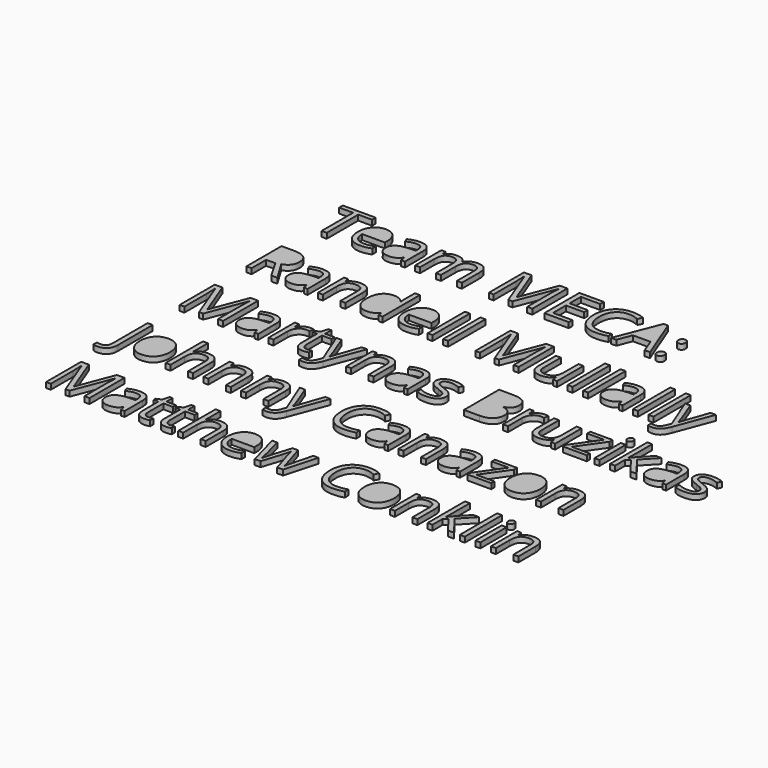
from build123d import *

# Parameters (mm, degrees)
F0_TEXT_SIZE = 6.9151809833
F1_DEPTH     = 0.6


# Not quite as in the source:
# - Text() gives the source's letters only with a copy of the font that has no kerning and outlines rounded to 1/6400 em; it was checked with that copy


with BuildPart() as f1:
    # F0 (on Top) → F1 (new body)
    with BuildSketch(Plane.XY):
        with BuildLine():
            add(Edge.make_bspline(
                [(5.8827660724, 1.8456028601), (5.6023770935, 1.484176604), (5.6023770935, 0.768887571)],
                knots=[0, 0, 0, 1, 1, 1], degree=2))
            add(Edge.make_bspline(
                [(5.6023770935, 0.768887571), (5.6023770935, 0.0590010232), (5.8860075635, -0.3121497061)],
                knots=[0, 0, 0, 1, 1, 1], degree=2))
            add(Edge.make_bspline(
                [(5.8860075635, -0.3121497061), (6.1696380335, -0.6833004355), (6.7196110211, -0.6833004355)],
                knots=[0, 0, 0, 1, 1, 1], degree=2))
            add(Edge.make_bspline(
                [(6.7196110211, -0.6833004355), (7.2706645057, -0.6833004355), (7.5559157212, -0.3137704517)],
                knots=[0, 0, 0, 1, 1, 1], degree=2))
            add(Edge.make_bspline(
                [(7.5559157212, -0.3137704517), (7.8411669368, 0.0557595321), (7.8411669368, 0.768887571)],
                knots=[0, 0, 0, 1, 1, 1], degree=2))
            add(Edge.make_bspline(
                [(7.8411669368, 0.768887571), (7.8411669368, 1.4744521307), (7.5559157212, 1.8407406234)],
                knots=[0, 0, 0, 1, 1, 1], degree=2))
            add(Edge.make_bspline(
                [(7.5559157212, 1.8407406234), (7.2706645057, 2.2070291161), (6.7131280389, 2.2070291161)],
                knots=[0, 0, 0, 1, 1, 1], degree=2))
            add(Edge.make_bspline(
                [(6.7131280389, 2.2070291161), (6.1631550513, 2.2070291161), (5.8827660724, 1.8456028601)],
                knots=[0, 0, 0, 1, 1, 1], degree=2))
        make_face()
        with BuildLine():
            add(Edge.make_bspline(
                [(14.8206374932, 11.2502489973), (14.5402485143, 10.8888227412), (14.5402485143, 10.1735337082)],
                knots=[0, 0, 0, 1, 1, 1], degree=2))
            add(Edge.make_bspline(
                [(14.5402485143, 10.1735337082), (14.5402485143, 9.4636471604), (14.8238789843, 9.0924964311)],
                knots=[0, 0, 0, 1, 1, 1], degree=2))
            add(Edge.make_bspline(
                [(14.8238789843, 9.0924964311), (15.1075094543, 8.7213457018), (15.6574824419, 8.7213457018)],
                knots=[0, 0, 0, 1, 1, 1], degree=2))
            add(Edge.make_bspline(
                [(15.6574824419, 8.7213457018), (16.2085359265, 8.7213457018), (16.4937871421, 9.0908756856)],
                knots=[0, 0, 0, 1, 1, 1], degree=2))
            add(Edge.make_bspline(
                [(16.4937871421, 9.0908756856), (16.7790383576, 9.4604056693), (16.7790383576, 10.1735337082)],
                knots=[0, 0, 0, 1, 1, 1], degree=2))
            add(Edge.make_bspline(
                [(16.7790383576, 10.1735337082), (16.7790383576, 10.8790982679), (16.4937871421, 11.2453867606)],
                knots=[0, 0, 0, 1, 1, 1], degree=2))
            add(Edge.make_bspline(
                [(16.4937871421, 11.2453867606), (16.2085359265, 11.6116752534), (15.6509994598, 11.6116752534)],
                knots=[0, 0, 0, 1, 1, 1], degree=2))
            add(Edge.make_bspline(
                [(15.6509994598, 11.6116752534), (15.1010264722, 11.6116752534), (14.8206374932, 11.2502489973)],
                knots=[0, 0, 0, 1, 1, 1], degree=2))
        make_face()
        with BuildLine():
            add(Edge.make_bspline(
                [(-26.9038357645, 11.2502489973), (-27.1842247434, 10.8888227412), (-27.1842247434, 10.1735337082)],
                knots=[0, 0, 0, 1, 1, 1], degree=2))
            add(Edge.make_bspline(
                [(-27.1842247434, 10.1735337082), (-27.1842247434, 9.4636471604), (-26.9005942734, 9.0924964311)],
                knots=[0, 0, 0, 1, 1, 1], degree=2))
            add(Edge.make_bspline(
                [(-26.9005942734, 9.0924964311), (-26.6169638033, 8.7213457018), (-26.0669908158, 8.7213457018)],
                knots=[0, 0, 0, 1, 1, 1], degree=2))
            add(Edge.make_bspline(
                [(-26.0669908158, 8.7213457018), (-25.5159373312, 8.7213457018), (-25.2306861156, 9.0908756856)],
                knots=[0, 0, 0, 1, 1, 1], degree=2))
            add(Edge.make_bspline(
                [(-25.2306861156, 9.0908756856), (-24.9454349001, 9.4604056693), (-24.9454349001, 10.1735337082)],
                knots=[0, 0, 0, 1, 1, 1], degree=2))
            add(Edge.make_bspline(
                [(-24.9454349001, 10.1735337082), (-24.9454349001, 10.8790982679), (-25.2306861156, 11.2453867606)],
                knots=[0, 0, 0, 1, 1, 1], degree=2))
            add(Edge.make_bspline(
                [(-25.2306861156, 11.2453867606), (-25.5159373312, 11.6116752534), (-26.0734737979, 11.6116752534)],
                knots=[0, 0, 0, 1, 1, 1], degree=2))
            add(Edge.make_bspline(
                [(-26.0734737979, 11.6116752534), (-26.6234467855, 11.6116752534), (-26.9038357645, 11.2502489973)],
                knots=[0, 0, 0, 1, 1, 1], degree=2))
        make_face()
        with BuildLine():
            add(Edge.make_bspline(
                [(-16.4068071313, 27.8920642323), (-16.1469475959, 27.5306379762), (-15.6434359806, 27.5306379762)],
                knots=[0, 0, 0, 1, 1, 1], degree=2))
            add(Edge.make_bspline(
                [(-15.6434359806, 27.5306379762), (-15.0696920583, 27.5306379762), (-14.8114532685, 27.8429016175)],
                knots=[0, 0, 0, 1, 1, 1], degree=2))
            add(Edge.make_bspline(
                [(-14.8114532685, 27.8429016175), (-14.5532144787, 28.1551652588), (-14.5532144787, 28.8510053452)],
                knots=[0, 0, 0, 1, 1, 1], degree=2))
            Line((-14.5532144787, 28.8510053452), (-14.5532144787, 28.9687795213))
            add(Edge.make_bspline(
                [(-14.5532144787, 28.9687795213), (-14.5532144787, 29.7553813582), (-14.8146947596, 30.0914159341)],
                knots=[0, 0, 0, 1, 1, 1], degree=2))
            add(Edge.make_bspline(
                [(-14.8146947596, 30.0914159341), (-15.0761750405, 30.42745051), (-15.6499189627, 30.42745051)],
                knots=[0, 0, 0, 1, 1, 1], degree=2))
            add(Edge.make_bspline(
                [(-15.6499189627, 30.42745051), (-16.1437061048, 30.42745051), (-16.4051863857, 30.0444143133)],
                knots=[0, 0, 0, 1, 1, 1], degree=2))
            add(Edge.make_bspline(
                [(-16.4051863857, 30.0444143133), (-16.6666666667, 29.6613781167), (-16.6666666667, 28.9622965391)],
                knots=[0, 0, 0, 1, 1, 1], degree=2))
            add(Edge.make_bspline(
                [(-16.6666666667, 28.9622965391), (-16.6666666667, 28.2534904884), (-16.4068071313, 27.8920642323)],
                knots=[0, 0, 0, 1, 1, 1], degree=2))
        make_face()
        with Locations((-30, 8.3194008071)):
            Text('Johnny Canazon', F0_TEXT_SIZE, font='Open Sans', text_align=(TextAlign.LEFT, TextAlign.BOTTOM))
        with BuildLine():
            Line((4.2582387898, 20.0611620173), (3.2749864938, 20.0611620173))
            Line((3.2749864938, 20.0611620173), (3.2749864938, 18.2135120983))
            Line((3.2749864938, 18.2135120983), (4.3057806591, 18.2135120983))
            add(Edge.make_bspline(
                [(4.3057806591, 18.2135120983), (4.9032955159, 18.2135120983), (5.2052944354, 18.4447384624)],
                knots=[0, 0, 0, 1, 1, 1], degree=2))
            add(Edge.make_bspline(
                [(5.2052944354, 18.4447384624), (5.5072933549, 18.6759648266), (5.5072933549, 19.1697519686)],
                knots=[0, 0, 0, 1, 1, 1], degree=2))
            add(Edge.make_bspline(
                [(5.5072933549, 19.1697519686), (5.5072933549, 19.6289632058), (5.1982712048, 19.8450626115)],
                knots=[0, 0, 0, 1, 1, 1], degree=2))
            add(Edge.make_bspline(
                [(5.1982712048, 19.8450626115), (4.8892490546, 20.0611620173), (4.2582387898, 20.0611620173)],
                knots=[0, 0, 0, 1, 1, 1], degree=2))
        make_face()
        with BuildLine():
            Line((-28.7477039438, 31.56197239), (-28.7477039438, 29.674344081))
            Line((-28.7477039438, 29.674344081), (-27.9600216099, 29.674344081))
            add(Edge.make_bspline(
                [(-27.9600216099, 29.674344081), (-27.3527822798, 29.674344081), (-27.0691518098, 29.9158351669)],
                knots=[0, 0, 0, 1, 1, 1], degree=2))
            add(Edge.make_bspline(
                [(-27.0691518098, 29.9158351669), (-26.7855213398, 30.1573262528), (-26.7855213398, 30.6403084246)],
                knots=[0, 0, 0, 1, 1, 1], degree=2))
            add(Edge.make_bspline(
                [(-26.7855213398, 30.6403084246), (-26.7855213398, 31.1297735786), (-27.0740140465, 31.3458729843)],
                knots=[0, 0, 0, 1, 1, 1], degree=2))
            add(Edge.make_bspline(
                [(-27.0740140465, 31.3458729843), (-27.3625067531, 31.56197239), (-28.001080497, 31.56197239)],
                knots=[0, 0, 0, 1, 1, 1], degree=2))
            Line((-28.001080497, 31.56197239), (-28.7477039438, 31.56197239))
        make_face()
        with BuildLine():
            Line((3.2749864938, 22.163809235), (3.2749864938, 20.5473856802))
            Line((3.2749864938, 20.5473856802), (4.2204213938, 20.5473856802))
            add(Edge.make_bspline(
                [(4.2204213938, 20.5473856802), (4.828741221, 20.5473856802), (5.095623987, 20.7380934057)],
                knots=[0, 0, 0, 1, 1, 1], degree=2))
            add(Edge.make_bspline(
                [(5.095623987, 20.7380934057), (5.3625067531, 20.9288011313), (5.3625067531, 21.3804488892)],
                knots=[0, 0, 0, 1, 1, 1], degree=2))
            add(Edge.make_bspline(
                [(5.3625067531, 21.3804488892), (5.3625067531, 21.7964402453), (5.0653700702, 21.9801247401)],
                knots=[0, 0, 0, 1, 1, 1], degree=2))
            add(Edge.make_bspline(
                [(5.0653700702, 21.9801247401), (4.7682333874, 22.163809235), (4.1199351702, 22.163809235)],
                knots=[0, 0, 0, 1, 1, 1], degree=2))
            Line((4.1199351702, 22.163809235), (3.2749864938, 22.163809235))
        make_face()
        with Locations((-30, 27.1286930816)):
            Text('Randell Mullally', F0_TEXT_SIZE, font='Open Sans', text_align=(TextAlign.LEFT, TextAlign.BOTTOM))
        with BuildLine():
            add(Edge.make_bspline(
                [(-21.2047541869, 37.087093946), (-21.0210696921, 36.9288011313), (-20.6904376013, 36.9288011313)],
                knots=[0, 0, 0, 1, 1, 1], degree=2))
            add(Edge.make_bspline(
                [(-20.6904376013, 36.9288011313), (-20.1663965424, 36.9288011313), (-19.867639114, 37.2156730924)],
                knots=[0, 0, 0, 1, 1, 1], degree=2))
            add(Edge.make_bspline(
                [(-19.867639114, 37.2156730924), (-19.5688816856, 37.5025450535), (-19.5688816856, 38.0190226331)],
                knots=[0, 0, 0, 1, 1, 1], degree=2))
            Line((-19.5688816856, 38.0190226331), (-19.5688816856, 38.352896215))
            Line((-19.5688816856, 38.352896215), (-20.1296596434, 38.3302057774))
            add(Edge.make_bspline(
                [(-20.1296596434, 38.3302057774), (-20.7984873042, 38.3064348428), (-21.093462993, 38.1222100994)],
                knots=[0, 0, 0, 1, 1, 1], degree=2))
            add(Edge.make_bspline(
                [(-21.093462993, 38.1222100994), (-21.3884386818, 37.937985356), (-21.3884386818, 37.5500869227)],
                knots=[0, 0, 0, 1, 1, 1], degree=2))
            add(Edge.make_bspline(
                [(-21.3884386818, 37.5500869227), (-21.3884386818, 37.2453867606), (-21.2047541869, 37.087093946)],
                knots=[0, 0, 0, 1, 1, 1], degree=2))
        make_face()
        with BuildLine():
            add(Edge.make_bspline(
                [(-24.6364127499, 27.6824478087), (-24.452728255, 27.524154994), (-24.1220961642, 27.524154994)],
                knots=[0, 0, 0, 1, 1, 1], degree=2))
            add(Edge.make_bspline(
                [(-24.1220961642, 27.524154994), (-23.5980551053, 27.524154994), (-23.2992976769, 27.8110269551)],
                knots=[0, 0, 0, 1, 1, 1], degree=2))
            add(Edge.make_bspline(
                [(-23.2992976769, 27.8110269551), (-23.0005402485, 28.0978989162), (-23.0005402485, 28.6143764959)],
                knots=[0, 0, 0, 1, 1, 1], degree=2))
            Line((-23.0005402485, 28.6143764959), (-23.0005402485, 28.9482500778))
            Line((-23.0005402485, 28.9482500778), (-23.5613182064, 28.9255596402))
            add(Edge.make_bspline(
                [(-23.5613182064, 28.9255596402), (-24.2301458671, 28.9017887055), (-24.5251215559, 28.7175639622)],
                knots=[0, 0, 0, 1, 1, 1], degree=2))
            add(Edge.make_bspline(
                [(-24.5251215559, 28.7175639622), (-24.8200972447, 28.5333392188), (-24.8200972447, 28.1454407855)],
                knots=[0, 0, 0, 1, 1, 1], degree=2))
            add(Edge.make_bspline(
                [(-24.8200972447, 28.1454407855), (-24.8200972447, 27.8407406234), (-24.6364127499, 27.6824478087)],
                knots=[0, 0, 0, 1, 1, 1], degree=2))
        make_face()
        with BuildLine():
            add(Edge.make_bspline(
                [(10.8525121556, 27.6824478087), (11.0361966505, 27.524154994), (11.3668287412, 27.524154994)],
                knots=[0, 0, 0, 1, 1, 1], degree=2))
            add(Edge.make_bspline(
                [(11.3668287412, 27.524154994), (11.8908698001, 27.524154994), (12.1896272285, 27.8110269551)],
                knots=[0, 0, 0, 1, 1, 1], degree=2))
            add(Edge.make_bspline(
                [(12.1896272285, 27.8110269551), (12.4883846569, 28.0978989162), (12.4883846569, 28.6143764959)],
                knots=[0, 0, 0, 1, 1, 1], degree=2))
            Line((12.4883846569, 28.6143764959), (12.4883846569, 28.9482500778))
            Line((12.4883846569, 28.9482500778), (11.9276066991, 28.9255596402))
            add(Edge.make_bspline(
                [(11.9276066991, 28.9255596402), (11.2587790384, 28.9017887055), (10.9638033495, 28.7175639622)],
                knots=[0, 0, 0, 1, 1, 1], degree=2))
            add(Edge.make_bspline(
                [(10.9638033495, 28.7175639622), (10.6688276607, 28.5333392188), (10.6688276607, 28.1454407855)],
                knots=[0, 0, 0, 1, 1, 1], degree=2))
            add(Edge.make_bspline(
                [(10.6688276607, 28.1454407855), (10.6688276607, 27.8407406234), (10.8525121556, 27.6824478087)],
                knots=[0, 0, 0, 1, 1, 1], degree=2))
        make_face()
        with BuildLine():
            add(Edge.make_bspline(
                [(-22.6677471637, 18.2778016715), (-22.4840626688, 18.1195088568), (-22.1534305781, 18.1195088568)],
                knots=[0, 0, 0, 1, 1, 1], degree=2))
            add(Edge.make_bspline(
                [(-22.1534305781, 18.1195088568), (-21.6293895192, 18.1195088568), (-21.3306320908, 18.4063808179)],
                knots=[0, 0, 0, 1, 1, 1], degree=2))
            add(Edge.make_bspline(
                [(-21.3306320908, 18.4063808179), (-21.0318746623, 18.693252779), (-21.0318746623, 19.2097303587)],
                knots=[0, 0, 0, 1, 1, 1], degree=2))
            Line((-21.0318746623, 19.2097303587), (-21.0318746623, 19.5436039406))
            Line((-21.0318746623, 19.5436039406), (-21.5926526202, 19.5209135029))
            add(Edge.make_bspline(
                [(-21.5926526202, 19.5209135029), (-22.2614802809, 19.4971425683), (-22.5564559697, 19.3129178249)],
                knots=[0, 0, 0, 1, 1, 1], degree=2))
            add(Edge.make_bspline(
                [(-22.5564559697, 19.3129178249), (-22.8514316586, 19.1286930816), (-22.8514316586, 18.7407946483)],
                knots=[0, 0, 0, 1, 1, 1], degree=2))
            add(Edge.make_bspline(
                [(-22.8514316586, 18.7407946483), (-22.8514316586, 18.4360944862), (-22.6677471637, 18.2778016715)],
                knots=[0, 0, 0, 1, 1, 1], degree=2))
        make_face()
        with BuildLine():
            add(Edge.make_bspline(
                [(-5.8292814695, 18.2778016715), (-5.6455969746, 18.1195088568), (-5.3149648838, 18.1195088568)],
                knots=[0, 0, 0, 1, 1, 1], degree=2))
            add(Edge.make_bspline(
                [(-5.3149648838, 18.1195088568), (-4.790923825, 18.1195088568), (-4.4921663965, 18.4063808179)],
                knots=[0, 0, 0, 1, 1, 1], degree=2))
            add(Edge.make_bspline(
                [(-4.4921663965, 18.4063808179), (-4.1934089681, 18.693252779), (-4.1934089681, 19.2097303587)],
                knots=[0, 0, 0, 1, 1, 1], degree=2))
            Line((-4.1934089681, 19.2097303587), (-4.1934089681, 19.5436039406))
            Line((-4.1934089681, 19.5436039406), (-4.754186926, 19.5209135029))
            add(Edge.make_bspline(
                [(-4.754186926, 19.5209135029), (-5.4230145867, 19.4971425683), (-5.7179902755, 19.3129178249)],
                knots=[0, 0, 0, 1, 1, 1], degree=2))
            add(Edge.make_bspline(
                [(-5.7179902755, 19.3129178249), (-6.0129659643, 19.1286930816), (-6.0129659643, 18.7407946483)],
                knots=[0, 0, 0, 1, 1, 1], degree=2))
            add(Edge.make_bspline(
                [(-6.0129659643, 18.7407946483), (-6.0129659643, 18.4360944862), (-5.8292814695, 18.2778016715)],
                knots=[0, 0, 0, 1, 1, 1], degree=2))
        make_face()
        with BuildLine():
            add(Edge.make_bspline(
                [(-0.5099945975, 8.8731555343), (-0.3263101026, 8.7148627196), (0.0043219881, 8.7148627196)],
                knots=[0, 0, 0, 1, 1, 1], degree=2))
            add(Edge.make_bspline(
                [(0.0043219881, 8.7148627196), (0.528363047, 8.7148627196), (0.8271204754, 9.0017346807)],
                knots=[0, 0, 0, 1, 1, 1], degree=2))
            add(Edge.make_bspline(
                [(0.8271204754, 9.0017346807), (1.1258779038, 9.2886066418), (1.1258779038, 9.8050842215)],
                knots=[0, 0, 0, 1, 1, 1], degree=2))
            Line((1.1258779038, 9.8050842215), (1.1258779038, 10.1389578033))
            Line((1.1258779038, 10.1389578033), (0.565099946, 10.1162673657))
            add(Edge.make_bspline(
                [(0.565099946, 10.1162673657), (-0.1037277147, 10.0924964311), (-0.3987034036, 9.9082716877)],
                knots=[0, 0, 0, 1, 1, 1], degree=2))
            add(Edge.make_bspline(
                [(-0.3987034036, 9.9082716877), (-0.6936790924, 9.7240469443), (-0.6936790924, 9.3361485111)],
                knots=[0, 0, 0, 1, 1, 1], degree=2))
            add(Edge.make_bspline(
                [(-0.6936790924, 9.3361485111), (-0.6936790924, 9.031448349), (-0.5099945975, 8.8731555343)],
                knots=[0, 0, 0, 1, 1, 1], degree=2))
        make_face()
        with BuildLine():
            add(Edge.make_bspline(
                [(7.5796866559, 8.8731555343), (7.7633711507, 8.7148627196), (8.0940032415, 8.7148627196)],
                knots=[0, 0, 0, 1, 1, 1], degree=2))
            add(Edge.make_bspline(
                [(8.0940032415, 8.7148627196), (8.6180443004, 8.7148627196), (8.9168017288, 9.0017346807)],
                knots=[0, 0, 0, 1, 1, 1], degree=2))
            add(Edge.make_bspline(
                [(8.9168017288, 9.0017346807), (9.2155591572, 9.2886066418), (9.2155591572, 9.8050842215)],
                knots=[0, 0, 0, 1, 1, 1], degree=2))
            Line((9.2155591572, 9.8050842215), (9.2155591572, 10.1389578033))
            Line((9.2155591572, 10.1389578033), (8.6547811994, 10.1162673657))
            add(Edge.make_bspline(
                [(8.6547811994, 10.1162673657), (7.9859535386, 10.0924964311), (7.6909778498, 9.9082716877)],
                knots=[0, 0, 0, 1, 1, 1], degree=2))
            add(Edge.make_bspline(
                [(7.6909778498, 9.9082716877), (7.396002161, 9.7240469443), (7.396002161, 9.3361485111)],
                knots=[0, 0, 0, 1, 1, 1], degree=2))
            add(Edge.make_bspline(
                [(7.396002161, 9.3361485111), (7.396002161, 9.031448349), (7.5796866559, 8.8731555343)],
                knots=[0, 0, 0, 1, 1, 1], degree=2))
        make_face()
        with BuildLine():
            add(Edge.make_bspline(
                [(23.2739059968, 18.2778016715), (23.4575904916, 18.1195088568), (23.7882225824, 18.1195088568)],
                knots=[0, 0, 0, 1, 1, 1], degree=2))
            add(Edge.make_bspline(
                [(23.7882225824, 18.1195088568), (24.3122636413, 18.1195088568), (24.6110210697, 18.4063808179)],
                knots=[0, 0, 0, 1, 1, 1], degree=2))
            add(Edge.make_bspline(
                [(24.6110210697, 18.4063808179), (24.9097784981, 18.693252779), (24.9097784981, 19.2097303587)],
                knots=[0, 0, 0, 1, 1, 1], degree=2))
            Line((24.9097784981, 19.2097303587), (24.9097784981, 19.5436039406))
            Line((24.9097784981, 19.5436039406), (24.3490005402, 19.5209135029))
            add(Edge.make_bspline(
                [(24.3490005402, 19.5209135029), (23.6801728795, 19.4971425683), (23.3851971907, 19.3129178249)],
                knots=[0, 0, 0, 1, 1, 1], degree=2))
            add(Edge.make_bspline(
                [(23.3851971907, 19.3129178249), (23.0902215019, 19.1286930816), (23.0902215019, 18.7407946483)],
                knots=[0, 0, 0, 1, 1, 1], degree=2))
            add(Edge.make_bspline(
                [(23.0902215019, 18.7407946483), (23.0902215019, 18.4360944862), (23.2739059968, 18.2778016715)],
                knots=[0, 0, 0, 1, 1, 1], degree=2))
        make_face()
        with BuildLine():
            add(Edge.make_bspline(
                [(-22.6677471637, -0.5314906029), (-22.4840626688, -0.6897834176), (-22.1534305781, -0.6897834176)],
                knots=[0, 0, 0, 1, 1, 1], degree=2))
            add(Edge.make_bspline(
                [(-22.1534305781, -0.6897834176), (-21.6293895192, -0.6897834176), (-21.3306320908, -0.4029114565)],
                knots=[0, 0, 0, 1, 1, 1], degree=2))
            add(Edge.make_bspline(
                [(-21.3306320908, -0.4029114565), (-21.0318746623, -0.1160394954), (-21.0318746623, 0.4004380843)],
                knots=[0, 0, 0, 1, 1, 1], degree=2))
            Line((-21.0318746623, 0.4004380843), (-21.0318746623, 0.7343116661))
            Line((-21.0318746623, 0.7343116661), (-21.5926526202, 0.7116212285))
            add(Edge.make_bspline(
                [(-21.5926526202, 0.7116212285), (-22.2614802809, 0.6878502939), (-22.5564559697, 0.5036255505)],
                knots=[0, 0, 0, 1, 1, 1], degree=2))
            add(Edge.make_bspline(
                [(-22.5564559697, 0.5036255505), (-22.8514316586, 0.3194008071), (-22.8514316586, -0.0684976262)],
                knots=[0, 0, 0, 1, 1, 1], degree=2))
            add(Edge.make_bspline(
                [(-22.8514316586, -0.0684976262), (-22.8514316586, -0.3731977882), (-22.6677471637, -0.5314906029)],
                knots=[0, 0, 0, 1, 1, 1], degree=2))
        make_face()
        with BuildLine():
            Line((5.623987034, 38.6197789811), (7.2209616424, 38.6197789811))
            Line((7.2209616424, 38.6197789811), (6.6461372231, 40.1497627736))
            add(Edge.make_bspline(
                [(6.6461372231, 40.1497627736), (6.5348460292, 40.4404164743), (6.4170718531, 40.8618103155)],
                knots=[0, 0, 0, 1, 1, 1], degree=2))
            add(Edge.make_bspline(
                [(6.4170718531, 40.8618103155), (6.3425175581, 40.5376612069), (6.2042139384, 40.1497627736)],
                knots=[0, 0, 0, 1, 1, 1], degree=2))
            Line((6.2042139384, 40.1497627736), (5.623987034, 38.6197789811))
        make_face()
        with BuildLine():
            add(Edge.make_bspline(
                [(-10.7169097785, 30.1454407855), (-10.9529983793, 30.42745051), (-11.3927606699, 30.42745051)],
                knots=[0, 0, 0, 1, 1, 1], degree=2))
            add(Edge.make_bspline(
                [(-11.3927606699, 30.42745051), (-11.8379254457, 30.42745051), (-12.1031874662, 30.1373370578)],
                knots=[0, 0, 0, 1, 1, 1], degree=2))
            add(Edge.make_bspline(
                [(-12.1031874662, 30.1373370578), (-12.3684494868, 29.8472236056), (-12.415991356, 29.333987517)],
                knots=[0, 0, 0, 1, 1, 1], degree=2))
            Line((-12.415991356, 29.333987517), (-10.4808211777, 29.333987517))
            add(Edge.make_bspline(
                [(-10.4808211777, 29.333987517), (-10.4808211777, 29.863431061), (-10.7169097785, 30.1454407855)],
                knots=[0, 0, 0, 1, 1, 1], degree=2))
        make_face()
        with BuildLine():
            add(Edge.make_bspline(
                [(-23.4927066451, 39.5500869227), (-23.7287952458, 39.8320966472), (-24.1685575365, 39.8320966472)],
                knots=[0, 0, 0, 1, 1, 1], degree=2))
            add(Edge.make_bspline(
                [(-24.1685575365, 39.8320966472), (-24.6137223123, 39.8320966472), (-24.8789843328, 39.541983195)],
                knots=[0, 0, 0, 1, 1, 1], degree=2))
            add(Edge.make_bspline(
                [(-24.8789843328, 39.541983195), (-25.1442463533, 39.2518697428), (-25.1917882226, 38.7386336542)],
                knots=[0, 0, 0, 1, 1, 1], degree=2))
            Line((-25.1917882226, 38.7386336542), (-23.2566180443, 38.7386336542))
            add(Edge.make_bspline(
                [(-23.2566180443, 38.7386336542), (-23.2566180443, 39.2680771982), (-23.4927066451, 39.5500869227)],
                knots=[0, 0, 0, 1, 1, 1], degree=2))
        make_face()
        with BuildLine():
            add(Edge.make_bspline(
                [(-8.1042679633, 1.9315023738), (-8.340356564, 2.2135120983), (-8.7801188547, 2.2135120983)],
                knots=[0, 0, 0, 1, 1, 1], degree=2))
            add(Edge.make_bspline(
                [(-8.7801188547, 2.2135120983), (-9.2252836305, 2.2135120983), (-9.490545651, 1.9233986461)],
                knots=[0, 0, 0, 1, 1, 1], degree=2))
            add(Edge.make_bspline(
                [(-9.490545651, 1.9233986461), (-9.7558076715, 1.6332851939), (-9.8033495408, 1.1200491053)],
                knots=[0, 0, 0, 1, 1, 1], degree=2))
            Line((-9.8033495408, 1.1200491053), (-7.8681793625, 1.1200491053))
            add(Edge.make_bspline(
                [(-7.8681793625, 1.1200491053), (-7.8681793625, 1.6494926494), (-8.1042679633, 1.9315023738)],
                knots=[0, 0, 0, 1, 1, 1], degree=2))
        make_face()
        with Locations((-30, 36.5333392188)):
            Text('Team MECA:', F0_TEXT_SIZE, font='Open Sans', text_align=(TextAlign.LEFT, TextAlign.BOTTOM))
        with Locations((-30, -1.0852453301)):
            Text('Matthew Conklin', F0_TEXT_SIZE, font='Open Sans', text_align=(TextAlign.LEFT, TextAlign.BOTTOM))
        with Locations((-30, 17.7240469443)):
            Text('Martynas Bruzikas', F0_TEXT_SIZE, font='Open Sans', text_align=(TextAlign.LEFT, TextAlign.BOTTOM))
    extrude(amount=F1_DEPTH)


solid = f1.part
